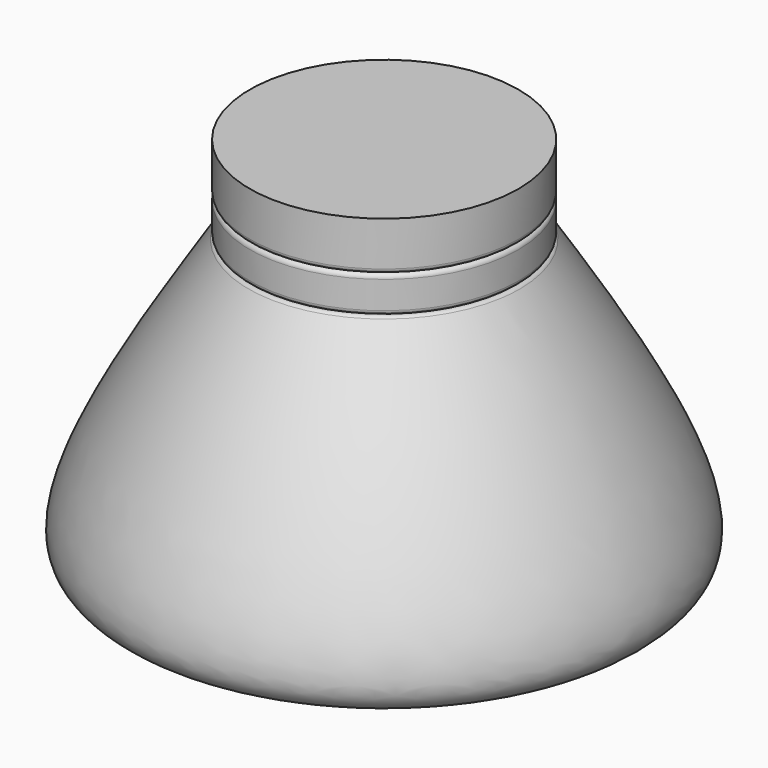
from build123d import *

# Parameters (mm, degrees)
F2_R = 1.49999


# Not quite as in the source:
# - a fillet or chamfer is up to 0.001 mm smaller than in the source, because OpenCascade refuses the exact size


with BuildPart() as f1:
    # F0 (on Front) → F1 (revolve)
    with BuildSketch(Plane.XZ):
        with BuildLine():
            Line((0, 0), (50, 0))
            add(Edge.make_bspline(
                [(44, 97), (63.5837763548, 66.2790611386), (106.3151142134, -0.7154386643), (69.4463568757, 0), (50, 0)],
                knots=[0, 0, 0, 0, 0.6178236159, 1, 1, 1, 1], degree=3))
            Line((44, 97), (41, 97))
            Line((41, 97), (41, 109))
            Line((41, 109), (44, 109))
            Line((44, 109), (44, 125))
            Line((44, 125), (0, 125))
            Line((0, 125), (0, 0))
        make_face()
    revolve(axis=Axis((0, 0, 62.5), (0, 0, 1)))

    # F2 (radius 1.5 in the source; OpenCascade refuses exactly that, so slightly less here)
    f2_edges = [f1.edges().sort_by_distance(p)[0] for p in [
        (-44, 0, 109),
        (-41, 0, 97),
        (-50, 0, 0),
        (-44, 0, 97),
        (78.864915, 0, 37.455621),
        (-41, 0, 109),
    ]]
    fillet(f2_edges, radius=F2_R)


with BuildPart() as f4:
    # F3 (on Front) → F4 (revolve)
    with BuildSketch(Plane.XZ):
        with BuildLine():
            Line((44, 98.5), (44, 107.5))
            ThreePointArc((44, 107.5), (42.5, 109), (41, 107.5))
            Line((41, 107.5), (41, 98.5))
            ThreePointArc((41, 98.5), (42.5, 97), (44, 98.5))
        make_face()
    revolve(axis=Axis((0, 0, 125), (0, 0, 1)))


solid = Compound([f1.part, f4.part])
